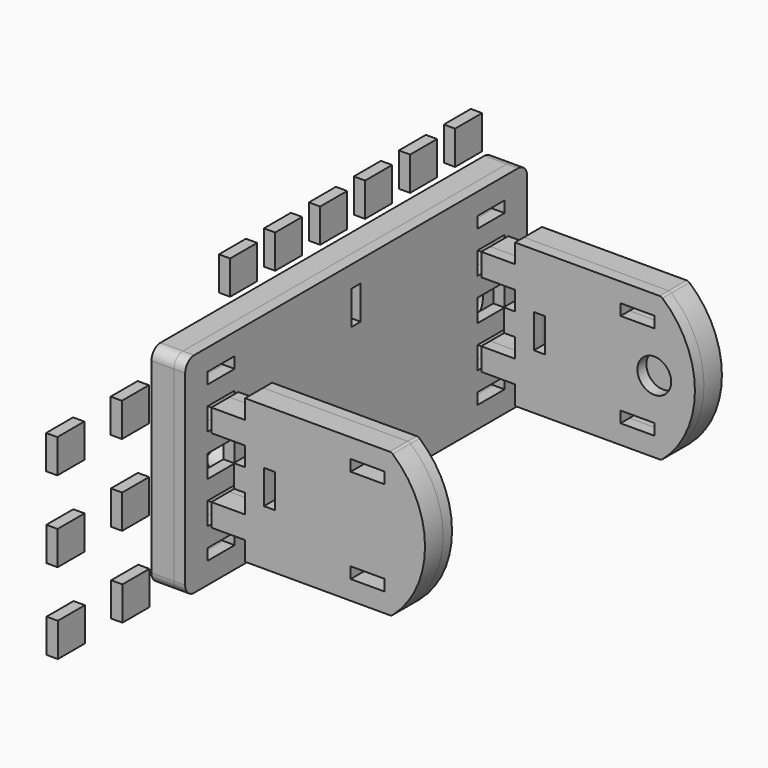
from build123d import *

# Parameters (mm, degrees)
F0_W     = 15
F0_H     = 5
F0_H_2   = 10
F0_W_2   = 5
F0_H_3   = 15
F1_DEPTH = 5
F2_DEPTH = 10
F4_W     = 15
F4_H     = 5
F4_W_2   = 5
F4_H_2   = 15
F4_R     = 7.5
F5_DEPTH = 5
F6_DEPTH = 10
F8_COUNT = 2


# Not quite as in the source:
# - a feature names something its author has since deleted; it is built from what else it names


with BuildPart() as f1:
    # F0 (on Right) → F1 (new body)
    with BuildSketch(Plane.YZ):
        with BuildLine():
            Line((-90, -46.5), (90, -46.5))
            ThreePointArc((90, -46.5), (93.5355339059, -45.0355339059), (95, -41.5))
            Line((95, -41.5), (95, 41.5))
            ThreePointArc((95, 41.5), (93.5355339059, 45.0355339059), (90, 46.5))
            Line((90, 46.5), (-90, 46.5))
            ThreePointArc((-90, 46.5), (-93.5355339059, 45.0355339059), (-95, 41.5))
            Line((-95, 41.5), (-95, -41.5))
            ThreePointArc((-95, -41.5), (-93.5355339059, -45.0355339059), (-90, -46.5))
        make_face()
        with Locations((-75, -34.5)):
            Rectangle(F0_W, F0_H, mode=Mode.SUBTRACT)
        with Locations((-75, -18.5)):
            Rectangle(F0_W, F0_H_2, mode=Mode.SUBTRACT)
        with BuildLine():
            ThreePointArc((-75.2821912081, 5), (-64.8945027994, 8.8754653026), (-58.25, 0))
            ThreePointArc((-58.25, 0), (-64.8945027994, -8.8754653026), (-75.2821912081, -5))
            Line((-75.2821912081, -5), (-82.5, -5))
            Line((-82.5, -5), (-82.5, 5))
            Line((-82.5, 5), (-75.2821912081, 5))
        make_face(mode=Mode.SUBTRACT)
        with Locations((0, -29.5)):
            Rectangle(F0_W_2, F0_H_3, mode=Mode.SUBTRACT)
        with Locations((75, -34.5)):
            Rectangle(F0_W, F0_H, mode=Mode.SUBTRACT)
        with Locations((75, -18.5)):
            Rectangle(F0_W, F0_H_2, mode=Mode.SUBTRACT)
        with BuildLine():
            ThreePointArc((75.2821912081, -5), (58.25, 0), (75.2821912081, 5))
            Line((75.2821912081, 5), (82.5, 5))
            Line((82.5, 5), (82.5, -5))
            Line((82.5, -5), (75.2821912081, -5))
        make_face(mode=Mode.SUBTRACT)
        with Locations((-75, 18.5)):
            Rectangle(F0_W, F0_H_2, mode=Mode.SUBTRACT)
        with Locations((-75, 34.5)):
            Rectangle(F0_W, F0_H, mode=Mode.SUBTRACT)
        with Locations((0, 29.5)):
            Rectangle(F0_W_2, F0_H_3, mode=Mode.SUBTRACT)
        with Locations((75, 18.5)):
            Rectangle(F0_W, F0_H_2, mode=Mode.SUBTRACT)
        with Locations((75, 34.5)):
            Rectangle(F0_W, F0_H, mode=Mode.SUBTRACT)
        with BuildLine():
            ThreePointArc((-75.2821912081, -5), (-64.8945027994, -8.8754653026), (-58.25, 0))
            ThreePointArc((-58.25, 0), (-64.8945027994, 8.8754653026), (-75.2821912081, 5))
            Line((-75.2821912081, 5), (-67.5, 5))
            Line((-67.5, 5), (-67.5, -5))
            Line((-67.5, -5), (-75.2821912081, -5))
        make_face()
        with BuildLine():
            Line((67.5, 5), (75.2821912081, 5))
            ThreePointArc((75.2821912081, 5), (58.25, 0), (75.2821912081, -5))
            Line((75.2821912081, -5), (67.5, -5))
            Line((67.5, -5), (67.5, 5))
        make_face()
    extrude(amount=F1_DEPTH)


with BuildPart() as f1b:
    # F0 (on Right) → F1, piece 2 (new body)
    with BuildSketch(Plane.YZ):
        with Locations((-158.5642143956, 37.8535165787)):
            Rectangle(F0_W, F0_H_3)
    extrude(amount=F1_DEPTH)


with BuildPart() as f1c:
    # F0 (on Right) → F1, piece 3 (new body)
    with BuildSketch(Plane.YZ):
        with Locations((-122.6688455811, 37.5)):
            Rectangle(F0_W, F0_H_3)
    extrude(amount=F1_DEPTH)


with BuildPart() as f1d:
    # F0 (on Right) → F1, piece 4 (new body)
    with BuildSketch(Plane.YZ):
        with Locations((-158.4228563942, 1.8537941087)):
            Rectangle(F0_W, F0_H_3)
    extrude(amount=F1_DEPTH)


with BuildPart() as f1e:
    # F0 (on Right) → F1, piece 5 (new body)
    with BuildSketch(Plane.YZ):
        with Locations((-122.5274875797, 1.50027753)):
            Rectangle(F0_W, F0_H_3)
    extrude(amount=F1_DEPTH)


with BuildPart() as f1f:
    # F0 (on Right) → F1, piece 6 (new body)
    with BuildSketch(Plane.YZ):
        with Locations((-158.2814983928, -34.1459283613)):
            Rectangle(F0_W, F0_H_3)
    extrude(amount=F1_DEPTH)


with BuildPart() as f1g:
    # F0 (on Right) → F1, piece 7 (new body)
    with BuildSketch(Plane.YZ):
        with Locations((-122.3861295783, -34.49944494)):
            Rectangle(F0_W, F0_H_3)
    extrude(amount=F1_DEPTH)


with BuildPart() as f1h:
    # F0 (on Right) → F1, piece 8 (new body)
    with BuildSketch(Plane.YZ):
        with Locations((-62.5, 68.7307228148)):
            Rectangle(F0_W, F0_H_3)
    extrude(amount=F1_DEPTH)


with BuildPart() as f1i:
    # F0 (on Right) → F1, piece 9 (new body)
    with BuildSketch(Plane.YZ):
        with Locations((-37.5, 68.7307228148)):
            Rectangle(F0_W, F0_H_3)
    extrude(amount=F1_DEPTH)


with BuildPart() as f1j:
    # F0 (on Right) → F1, piece 10 (new body)
    with BuildSketch(Plane.YZ):
        with Locations((-12.5, 68.7307228148)):
            Rectangle(F0_W, F0_H_3)
    extrude(amount=F1_DEPTH)


with BuildPart() as f1k:
    # F0 (on Right) → F1, piece 11 (new body)
    with BuildSketch(Plane.YZ):
        with Locations((12.5, 68.7307228148)):
            Rectangle(F0_W, F0_H_3)
    extrude(amount=F1_DEPTH)


with BuildPart() as f1l:
    # F0 (on Right) → F1, piece 12 (new body)
    with BuildSketch(Plane.YZ):
        with Locations((37.5, 68.7307228148)):
            Rectangle(F0_W, F0_H_3)
    extrude(amount=F1_DEPTH)


with BuildPart() as f1m:
    # F0 (on Right) → F1, piece 13 (new body)
    with BuildSketch(Plane.YZ):
        with Locations((62.5, 68.7307228148)):
            Rectangle(F0_W, F0_H_3)
    extrude(amount=F1_DEPTH)


with BuildPart() as f2:
    # F0 (on Right) → F2 (new body)
    with BuildSketch(Plane.YZ):
        with BuildLine():
            Line((-90, -46.5), (90, -46.5))
            ThreePointArc((90, -46.5), (93.5355339059, -45.0355339059), (95, -41.5))
            Line((95, -41.5), (95, 41.5))
            ThreePointArc((95, 41.5), (93.5355339059, 45.0355339059), (90, 46.5))
            Line((90, 46.5), (-90, 46.5))
            ThreePointArc((-90, 46.5), (-93.5355339059, 45.0355339059), (-95, 41.5))
            Line((-95, 41.5), (-95, -41.5))
            ThreePointArc((-95, -41.5), (-93.5355339059, -45.0355339059), (-90, -46.5))
        make_face()
        with Locations((-75, -34.5)):
            Rectangle(F0_W, F0_H, mode=Mode.SUBTRACT)
        with Locations((-75, -18.5)):
            Rectangle(F0_W, F0_H_2, mode=Mode.SUBTRACT)
        with BuildLine():
            ThreePointArc((-75.2821912081, 5), (-64.8945027994, 8.8754653026), (-58.25, 0))
            ThreePointArc((-58.25, 0), (-64.8945027994, -8.8754653026), (-75.2821912081, -5))
            Line((-75.2821912081, -5), (-82.5, -5))
            Line((-82.5, -5), (-82.5, 5))
            Line((-82.5, 5), (-75.2821912081, 5))
        make_face(mode=Mode.SUBTRACT)
        with Locations((0, -29.5)):
            Rectangle(F0_W_2, F0_H_3, mode=Mode.SUBTRACT)
        with Locations((75, -34.5)):
            Rectangle(F0_W, F0_H, mode=Mode.SUBTRACT)
        with Locations((75, -18.5)):
            Rectangle(F0_W, F0_H_2, mode=Mode.SUBTRACT)
        with BuildLine():
            ThreePointArc((75.2821912081, -5), (58.25, 0), (75.2821912081, 5))
            Line((75.2821912081, 5), (82.5, 5))
            Line((82.5, 5), (82.5, -5))
            Line((82.5, -5), (75.2821912081, -5))
        make_face(mode=Mode.SUBTRACT)
        with Locations((-75, 18.5)):
            Rectangle(F0_W, F0_H_2, mode=Mode.SUBTRACT)
        with Locations((-75, 34.5)):
            Rectangle(F0_W, F0_H, mode=Mode.SUBTRACT)
        with Locations((0, 29.5)):
            Rectangle(F0_W_2, F0_H_3, mode=Mode.SUBTRACT)
        with Locations((75, 18.5)):
            Rectangle(F0_W, F0_H_2, mode=Mode.SUBTRACT)
        with Locations((75, 34.5)):
            Rectangle(F0_W, F0_H, mode=Mode.SUBTRACT)
        with BuildLine():
            ThreePointArc((75.2821912081, 5), (76.3754653026, 2.6054972006), (76.75, 0))
            ThreePointArc((76.75, 0), (76.3754653026, -2.6054972006), (75.2821912081, -5))
            Line((75.2821912081, -5), (82.5, -5))
            Line((82.5, -5), (82.5, 5))
            Line((82.5, 5), (75.2821912081, 5))
        make_face()
        with BuildLine():
            ThreePointArc((-75.2821912081, -5), (-76.75, 0), (-75.2821912081, 5))
            Line((-75.2821912081, 5), (-82.5, 5))
            Line((-82.5, 5), (-82.5, -5))
            Line((-82.5, -5), (-75.2821912081, -5))
        make_face()
    extrude(amount=-F2_DEPTH)


with BuildPart() as f5:
    # F4 (on offset) → F5 (new body)
    with BuildSketch(Plane.XZ.offset(72.5)):
        with BuildLine():
            ThreePointArc((87.2068003959, 31.5138772077), (86.597053465, 31.8745338641), (85.8998283993, 32))
            Line((85.8998283993, 32), (21.6333333333, 32))
            Line((21.6333333333, 32), (21.6333333333, 23.5))
            Line((21.6333333333, 23.5), (6.6333333333, 23.5))
            Line((6.6333333333, 23.5), (6.6333333333, 13.5))
            Line((6.6333333333, 13.5), (21.6333333333, 13.5))
            Line((21.6333333333, 13.5), (21.6333333333, 5))
            Line((21.6333333333, 5), (16.6333333333, 5))
            Line((16.6333333333, 5), (16.6333333333, -5))
            Line((16.6333333333, -5), (21.6333333333, -5))
            Line((21.6333333333, -5), (21.6333333333, -13.5))
            Line((21.6333333333, -13.5), (6.6333333333, -13.5))
            Line((6.6333333333, -13.5), (6.6333333333, -23.5))
            Line((6.6333333333, -23.5), (21.6333333333, -23.5))
            Line((21.6333333333, -23.5), (21.6333333333, -32))
            Line((21.6333333333, -32), (85.8998283993, -32))
            ThreePointArc((85.8998283993, -32), (86.597053465, -31.8745338641), (87.2068003959, -31.5138772077))
            ThreePointArc((87.2068003959, -31.5138772077), (101.6333333333, 0), (87.2068003959, 31.5138772077))
        make_face()
        with Locations((76.0636103153, -21)):
            Rectangle(F4_W, F4_H, mode=Mode.SUBTRACT)
        with Locations((32.5, 0)):
            Rectangle(F4_W_2, F4_H_2, mode=Mode.SUBTRACT)
        with Locations((83.5636103153, 0)):
            Circle(F4_R, mode=Mode.SUBTRACT)
        with Locations((76.0636103153, 21)):
            Rectangle(F4_W, F4_H, mode=Mode.SUBTRACT)
    extrude(amount=-F5_DEPTH)


with BuildPart() as f6:
    # F4 (on offset) → F6 (new body)
    with BuildSketch(Plane.XZ.offset(72.5)):
        with BuildLine():
            ThreePointArc((87.2068003959, 31.5138772077), (86.597053465, 31.8745338641), (85.8998283993, 32))
            Line((85.8998283993, 32), (21.6333333333, 32))
            Line((21.6333333333, 32), (21.6333333333, 23.5))
            Line((21.6333333333, 23.5), (6.6333333333, 23.5))
            Line((6.6333333333, 23.5), (6.6333333333, 13.5))
            Line((6.6333333333, 13.5), (21.6333333333, 13.5))
            Line((21.6333333333, 13.5), (21.6333333333, 5))
            Line((21.6333333333, 5), (16.6333333333, 5))
            Line((16.6333333333, 5), (16.6333333333, -5))
            Line((16.6333333333, -5), (21.6333333333, -5))
            Line((21.6333333333, -5), (21.6333333333, -13.5))
            Line((21.6333333333, -13.5), (6.6333333333, -13.5))
            Line((6.6333333333, -13.5), (6.6333333333, -23.5))
            Line((6.6333333333, -23.5), (21.6333333333, -23.5))
            Line((21.6333333333, -23.5), (21.6333333333, -32))
            Line((21.6333333333, -32), (85.8998283993, -32))
            ThreePointArc((85.8998283993, -32), (86.597053465, -31.8745338641), (87.2068003959, -31.5138772077))
            ThreePointArc((87.2068003959, -31.5138772077), (101.6333333333, 0), (87.2068003959, 31.5138772077))
        make_face()
        with Locations((76.0636103153, -21)):
            Rectangle(F4_W, F4_H, mode=Mode.SUBTRACT)
        with Locations((32.5, 0)):
            Rectangle(F4_W_2, F4_H_2, mode=Mode.SUBTRACT)
        with Locations((83.5636103153, 0)):
            Circle(F4_R, mode=Mode.SUBTRACT)
        with Locations((76.0636103153, 21)):
            Rectangle(F4_W, F4_H, mode=Mode.SUBTRACT)
        with Locations((83.5636103153, 0)):
            Circle(F4_R)
    extrude(amount=F6_DEPTH)


with BuildPart() as f8_1:
    # F8: instance of F5
    add(f5.part.rotate(Axis((79.9781307578, 0, 0), (1, 0, 0)), 1 * 360 / F8_COUNT))


with BuildPart() as f8_2:
    # F8: instance of F6
    add(f6.part.rotate(Axis((79.9781307578, 0, 0), (1, 0, 0)), 1 * 360 / F8_COUNT))


solid = Compound([f1.part, f1b.part, f1c.part, f1d.part, f1e.part, f1f.part, f1g.part, f1h.part, f1i.part, f1j.part, f1k.part, f1l.part, f1m.part, f2.part, f5.part, f6.part, f8_1.part, f8_2.part])
